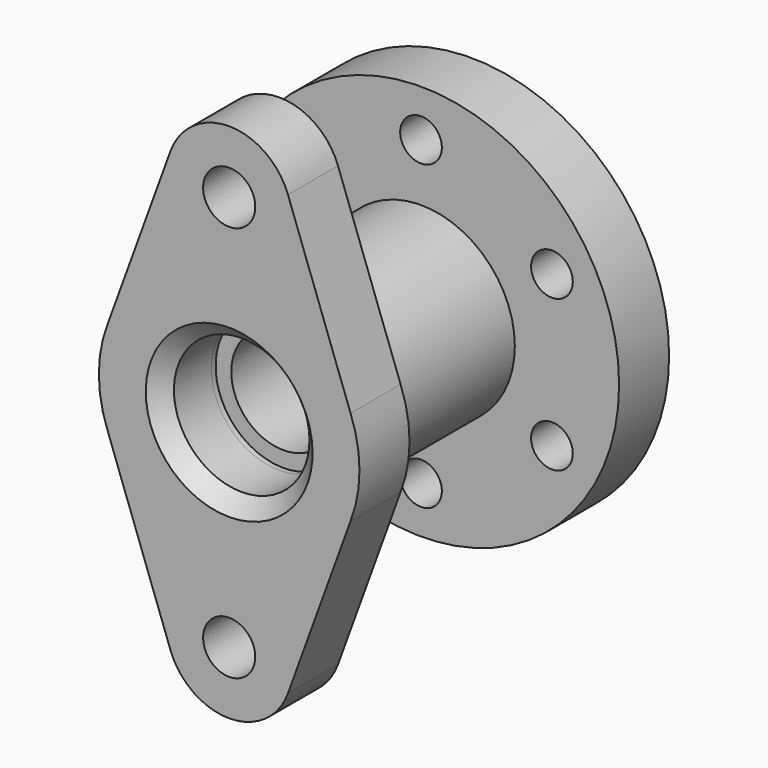
from build123d import *
from build123d import SkipClean  # not in build123d's __all__

# Parameters (mm, degrees)
F0_R     = 965.2
F0_R_2   = 101.6
F0_R_3   = 457.2
F1_DEPTH = 304.8
F0_R_4   = 330.2
F2_DEPTH = 1168.4
F0_R_5   = 254
F3_DEPTH = 1143
F5_DEPTH = 304.8
F6_SIZE2 = 76.2
F6_SIZE  = 76.2


# Not quite as in the source:
# - a feature names something its author has since deleted; it is built from what else it names


with BuildPart() as f1:
    # F0 (on Front) → F1 (new body)
    with BuildSketch(Plane.XZ):
        Circle(F0_R)
        with Locations((-637.9143124276, -368.3)):
            Circle(F0_R_2, mode=Mode.SUBTRACT)
        with Locations((0, -736.6)):
            Circle(F0_R_2, mode=Mode.SUBTRACT)
        with Locations((637.9143124276, -368.3)):
            Circle(F0_R_2, mode=Mode.SUBTRACT)
        with Locations((-637.9143124276, 368.3)):
            Circle(F0_R_2, mode=Mode.SUBTRACT)
        Circle(F0_R_3, mode=Mode.SUBTRACT)
        with Locations((637.9143124276, 368.3)):
            Circle(F0_R_2, mode=Mode.SUBTRACT)
        with Locations((0, 736.6)):
            Circle(F0_R_2, mode=Mode.SUBTRACT)
    extrude(amount=F1_DEPTH)

    # F0 (on Front) → F2 (join)
    with BuildSketch(Plane.XZ):
        Circle(F0_R_3)
        Circle(F0_R_4, mode=Mode.SUBTRACT)
    extrude(amount=F2_DEPTH)

    # F0 (on Front) → F3 (join)
    with BuildSketch(Plane.XZ):
        Circle(F0_R_4)
        Circle(F0_R_5, mode=Mode.SUBTRACT)
    extrude(amount=F3_DEPTH)

    # F4 (on face) → F5 (join)
    with BuildSketch(Plane.XZ.offset(1168.4)):
        with BuildLine():
            ThreePointArc((591.503767336, -230.9724945255), (624.031206054, -117.5161855696), (635, 0))
            ThreePointArc((635, 0), (624.031206054, 117.5161855696), (591.503767336, 230.9724945255))
            ThreePointArc((591.503767336, 230.9724945255), (358.1602057574, 524.3531891882), (0, 635))
            Line((0, 635), (0, 457.2))
            ThreePointArc((0, 457.2), (323.2892203585, 323.2892203585), (457.2, 0))
            ThreePointArc((457.2, 0), (323.2892203585, -323.2892203585), (0, -457.2))
            Line((0, -457.2), (0, -635))
            ThreePointArc((0, -635), (358.1602057574, -524.3531891882), (591.503767336, -230.9724945255))
        make_face()
        with BuildLine():
            ThreePointArc((0, 635), (358.1602057574, 524.3531891882), (591.503767336, 230.9724945255))
            Line((591.503767336, 230.9724945255), (286.428692972, 1069.4192105246))
            ThreePointArc((286.428692972, 1069.4192105246), (300.172038686, 1018.1130153278), (304.8, 965.2))
            ThreePointArc((304.8, 965.2), (215.5261469057, 749.6738530943), (0, 660.4))
            Line((0, 660.4), (0, 635))
        make_face()
        with BuildLine():
            Line((286.428692972, -1069.4192105246), (591.503767336, -230.9724945255))
            ThreePointArc((591.503767336, -230.9724945255), (358.1602057574, -524.3531891882), (0, -635))
            Line((0, -635), (0, -660.4))
            ThreePointArc((0, -660.4), (215.5261469057, -749.6738530943), (304.8, -965.2))
            ThreePointArc((304.8, -965.2), (300.172038686, -1018.1130153278), (286.428692972, -1069.4192105246))
        make_face()
        with BuildLine():
            Line((0, 457.2), (0, 635))
            ThreePointArc((0, 635), (-358.1602057574, 524.3531891882), (-591.503767336, 230.9724945255))
            ThreePointArc((-591.503767336, 230.9724945255), (-635, 0), (-591.503767336, -230.9724945255))
            ThreePointArc((-591.503767336, -230.9724945255), (-358.1602057574, -524.3531891882), (0, -635))
            Line((0, -635), (0, -457.2))
            ThreePointArc((0, -457.2), (-457.2, 0), (0, 457.2))
        make_face()
        with BuildLine():
            ThreePointArc((-591.503767336, 230.9724945255), (-358.1602057574, 524.3531891882), (0, 635))
            Line((0, 635), (0, 660.4))
            ThreePointArc((0, 660.4), (-249.6688360288, 790.3614678738), (-286.428692972, 1069.4192105246))
            Line((-286.428692972, 1069.4192105246), (-591.503767336, 230.9724945255))
        make_face()
        with BuildLine():
            ThreePointArc((304.8, 965.2), (300.172038686, 1018.1130153278), (286.428692972, 1069.4192105246))
            ThreePointArc((286.428692972, 1069.4192105246), (0, 1270), (-286.428692972, 1069.4192105246))
            ThreePointArc((-286.428692972, 1069.4192105246), (-249.6688360288, 790.3614678738), (0, 660.4))
            ThreePointArc((0, 660.4), (215.5261469057, 749.6738530943), (304.8, 965.2))
        make_face()
        with BuildLine():
            ThreePointArc((127, 965.2), (89.8025612107, 875.3974387893), (0, 838.2))
            ThreePointArc((0, 838.2), (-89.8025612107, 1055.0025612107), (127, 965.2))
        make_face(mode=Mode.SUBTRACT)
        with BuildLine():
            Line((0, -660.4), (0, -635))
            ThreePointArc((0, -635), (-358.1602057574, -524.3531891882), (-591.503767336, -230.9724945255))
            Line((-591.503767336, -230.9724945255), (-286.428692972, -1069.4192105246))
            ThreePointArc((-286.428692972, -1069.4192105246), (-249.6688360288, -790.3614678738), (0, -660.4))
        make_face()
        with BuildLine():
            ThreePointArc((-286.428692972, -1069.4192105246), (0, -1270), (286.428692972, -1069.4192105246))
            ThreePointArc((286.428692972, -1069.4192105246), (300.172038686, -1018.1130153278), (304.8, -965.2))
            ThreePointArc((304.8, -965.2), (215.5261469057, -749.6738530943), (0, -660.4))
            ThreePointArc((0, -660.4), (-249.6688360288, -790.3614678738), (-286.428692972, -1069.4192105246))
        make_face()
        with BuildLine():
            ThreePointArc((127, -965.2), (-89.8025612107, -1055.0025612107), (0, -838.2))
            ThreePointArc((0, -838.2), (89.8025612107, -875.3974387893), (127, -965.2))
        make_face(mode=Mode.SUBTRACT)
        with BuildLine():
            ThreePointArc((457.2, 0), (323.2892203585, 323.2892203585), (0, 457.2))
            Line((0, 457.2), (0, 330.2))
            ThreePointArc((0, 330.2), (233.4866591478, 233.4866591478), (330.2, 0))
            ThreePointArc((330.2, 0), (233.4866591478, -233.4866591478), (0, -330.2))
            Line((0, -330.2), (0, -457.2))
            ThreePointArc((0, -457.2), (323.2892203585, -323.2892203585), (457.2, 0))
        make_face()
        with BuildLine():
            Line((0, 330.2), (0, 457.2))
            ThreePointArc((0, 457.2), (-457.2, 0), (0, -457.2))
            Line((0, -457.2), (0, -330.2))
            ThreePointArc((0, -330.2), (-330.2, 0), (0, 330.2))
        make_face()
    with SkipClean():  # cleaning this boolean's faces spoils the solid; the shape is the same uncleaned
        extrude(amount=F5_DEPTH)

    # F6
    f6_edges = [f1.edges().sort_by_distance(p)[0] for p in [
        (0, -1473.2, 330.2),
    ]]
    chamfer(f6_edges, length=F6_SIZE, length2=F6_SIZE2)


solid = f1.part
